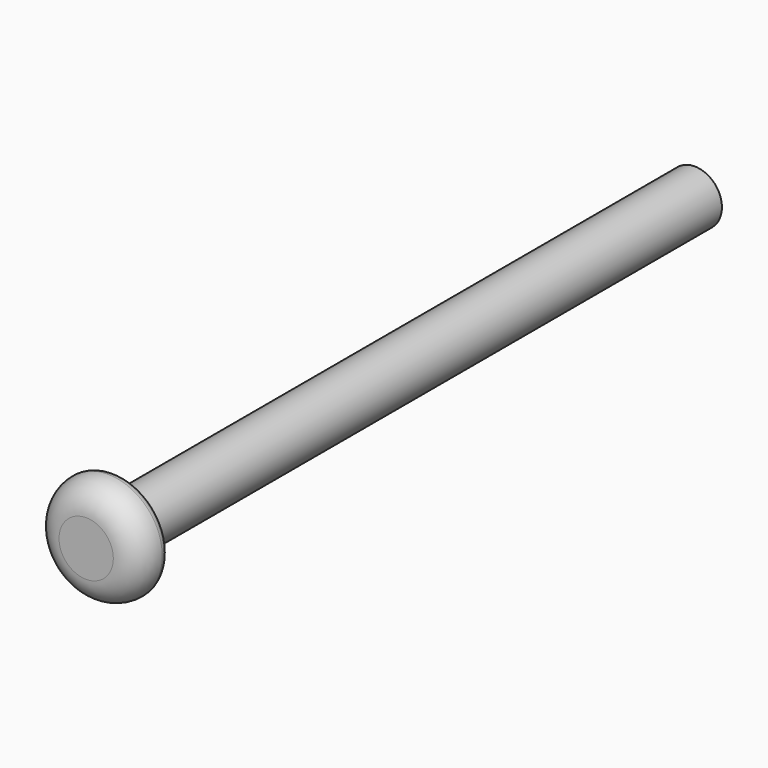
from build123d import *

# Parameters (mm, degrees)
F0_R     = 1.5
F1_DEPTH = 40
F2_R     = 3
F3_DEPTH = 2
F4_R     = 1.5
F5_R     = 0.49999


# Not quite as in the source:
# - a fillet or chamfer is up to 0.001 mm smaller than in the source, because OpenCascade refuses the exact size


with BuildPart() as f1:
    # F0 (on Front) → F1 (new body)
    with BuildSketch(Plane.XZ):
        Circle(F0_R)
    extrude(amount=-F1_DEPTH)

    # F2 (on face) → F3 (join)
    with BuildSketch(Plane.XZ):
        Circle(F2_R)
    extrude(amount=F3_DEPTH)

    # F4
    f4_edges = [f1.edges().sort_by_distance(p)[0] for p in [
        (-3, -2, 0),
    ]]
    fillet(f4_edges, radius=F4_R)

    # F5 (radius 0.5 in the source; OpenCascade refuses exactly that, so slightly less here)
    f5_edges = [f1.edges().sort_by_distance(p)[0] for p in [
        (-3, 0, 0),
    ]]
    fillet(f5_edges, radius=F5_R)


solid = f1.part
